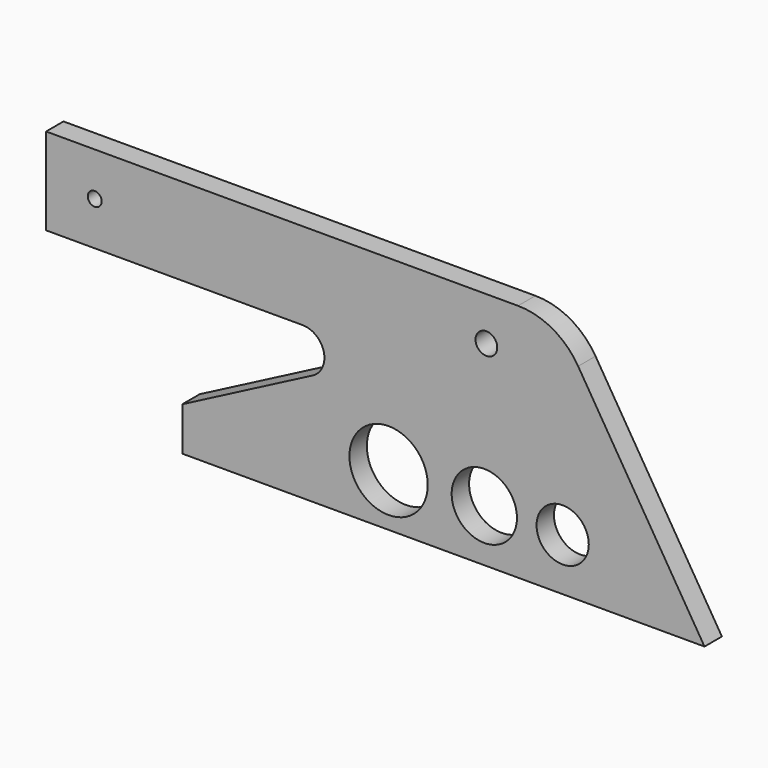
from build123d import *

# Parameters (mm, degrees)
F0_R        = 9
F0_R_2      = 7.5
F0_R_3      = 6
F0_R_4      = 1.6
F0_R_5      = 2.5
F1_DEPTH    = 5
F2_T1_DEPTH = 5


# Not quite as in the source:
# - a fillet or chamfer that OpenCascade refuses, or shapes differently, is made with other operations: its cross-section is extruded or revolved along the edge and cut away or added


with BuildPart() as f1:
    # F0 (on Front) → F1 (new body)
    with BuildSketch(Plane.XZ):
        with BuildLine():
            Line((77.14561722, 20), (-0.2484538774, 20))
            Line((-0.2484538774, 20), (-29.0604767571, 20))
            Line((-29.0604767571, 20), (-31.3025846086, 20))
            Line((-31.3025846086, 20), (-31.3025846086, 0))
            Line((-31.3025846086, 0), (0, 0))
            Line((0, 0), (33.9829302539, 0))
            ThreePointArc((33.9829302539, 0), (34.7117105365, -4.7760782671), (31.6838696315, -8.540945299))
            Line((31.6838696315, -8.540945299), (0, -25))
            Line((0, -25), (0, -35))
            Line((0, -35), (120, -35))
            Line((120, -35), (90.9631787703, 12.2713973983))
            ThreePointArc((90.9631787703, 12.2713973983), (85.0616816679, 17.9365681271), (77.14561722, 20))
        make_face()
        with Locations((47.4024499138, -23)):
            Circle(F0_R, mode=Mode.SUBTRACT)
        with Locations((69.4024499138, -23)):
            Circle(F0_R_2, mode=Mode.SUBTRACT)
        with Locations((87.4024499138, -23)):
            Circle(F0_R_3, mode=Mode.SUBTRACT)
        with Locations((-20.1252056134, 10)):
            Circle(F0_R_4, mode=Mode.SUBTRACT)
        with Locations((69.8747943866, 10)):
            Circle(F0_R_5, mode=Mode.SUBTRACT)
    extrude(amount=F1_DEPTH)

    # F2: fillet of radius 5 on 2 edges, made by hand

    # F2_s2 → F2_t1 (join)
    with BuildSketch(Plane.XZ):
        with BuildLine():
            ThreePointArc((29.9588910165, -9.4370327313), (32.5111722793, -3.8136534352), (27.6539527219, 0))
            Line((27.6539527219, 0), (27.6539527219, 0.5))
            Line((27.6539527219, 0.5), (33.9829302539, 0.5))
            Line((33.9829302539, 0.5), (34.4050124686, 0.2680421685))
            ThreePointArc((34.4050124686, 0.2680421685), (31.914363461, -8.9846485721), (30.189384846, -9.8807360044))
            Line((30.189384846, -9.8807360044), (29.9588910165, -9.4370327313))
        make_face()
    extrude(amount=F2_T1_DEPTH)


solid = f1.part
